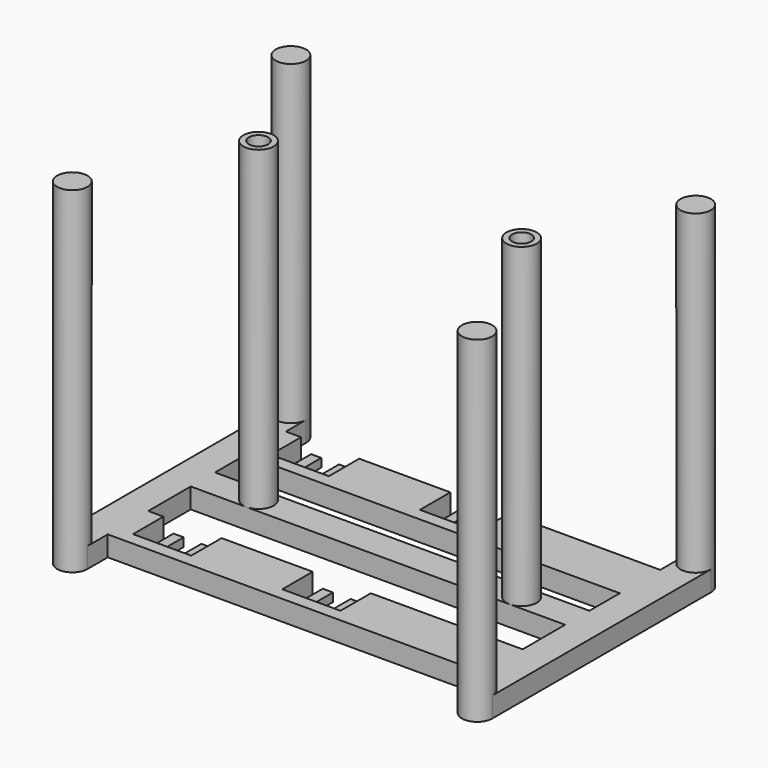
from build123d import *

# Parameters (mm, degrees)
F1_DEPTH  = 4
F2_W      = 2
F2_H      = 7.5
F3_DEPTH  = 1.7
F5_DEPTH  = 62.5
F4_R      = 3
F7_W      = 74
F7_H      = 6
F8_DEPTH  = 4
F9_R      = 1.9
F10_R     = 1.9
F11_DEPTH = 25


with BuildPart() as f1:
    # F0 (on Top) → F1 (new body)
    with BuildSketch(Plane.XY):
        with BuildLine():
            Line((6, 0), (80, 0))
            Line((80, 0), (80, -24))
            Line((80, -24), (80, -34))
            Line((80, -34), (80, -39))
            ThreePointArc((80, -39), (83, -42), (86, -39))
            Line((86, -39), (86, 15))
            ThreePointArc((86, 15), (83, 18), (80, 15))
            Line((80, 15), (80, 10))
            Line((80, 10), (50, 10))
            Line((50, 10), (50, 2.5))
            Line((50, 2.5), (38.5, 2.5))
            Line((38.5, 2.5), (38.5, 10))
            Line((38.5, 10), (20.5, 10))
            Line((20.5, 10), (20.5, 2.5))
            Line((20.5, 2.5), (9, 2.5))
            Line((9, 2.5), (9, 10))
            Line((9, 10), (6, 10))
            Line((6, 10), (6, 15))
            ThreePointArc((6, 15), (3, 18), (0, 15))
            Line((0, 15), (0, -39))
            ThreePointArc((0, -39), (3, -42), (6, -39))
            Line((6, -39), (6, -34))
            Line((6, -34), (6, -24))
            Line((6, -24), (6, 0))
        make_face()
        Polygon((80, -34), (80, -24), (50, -24), (50, -31.5), (38.5, -31.5), (38.5, -24), (20.5, -24), (20.5, -31.5), (9, -31.5), (9, -24), (6, -24), (6, -34), align=None)
    extrude(amount=F1_DEPTH)

    # F2 (on Top) → F3 (join)
    with BuildSketch(Plane.XY):
        with Locations((12, 6.25)):
            Rectangle(F2_W, F2_H)
        with Locations((17.5, 6.25)):
            Rectangle(F2_W, F2_H)
        with Locations((41.5, 6.25)):
            Rectangle(F2_W, F2_H)
        with Locations((47, 6.25)):
            Rectangle(F2_W, F2_H)
        with Locations((12, -27.75)):
            Rectangle(F2_W, F2_H)
        with Locations((17.5, -27.75)):
            Rectangle(F2_W, F2_H)
        with Locations((41.5, -27.75)):
            Rectangle(F2_W, F2_H)
        with Locations((47, -27.75)):
            Rectangle(F2_W, F2_H)
    extrude(amount=F3_DEPTH)

    # F4 (on face) → F5 (join)
    with BuildSketch(Plane.XY.offset(4)):
        with BuildLine():
            ThreePointArc((0, 15), (3, 12), (6, 15))
            ThreePointArc((6, 15), (3, 18), (0, 15))
        make_face()
        with BuildLine():
            ThreePointArc((6, -39), (3, -36), (0, -39))
            ThreePointArc((0, -39), (3, -42), (6, -39))
        make_face()
        with BuildLine():
            ThreePointArc((86, -39), (83, -36), (80, -39))
            ThreePointArc((80, -39), (83, -42), (86, -39))
        make_face()
        with BuildLine():
            ThreePointArc((80, 15), (83, 12), (86, 15))
            ThreePointArc((86, 15), (83, 18), (80, 15))
        make_face()
    extrude(amount=F5_DEPTH)



with BuildPart() as f5:
    # F4 (on face) → F5, piece 2 (new body)
    with BuildSketch(Plane.XY.offset(4)):
        with Locations((17, -10.5)):
            Circle(F4_R)
    extrude(amount=F5_DEPTH)


with BuildPart() as f5b:
    # F4 (on face) → F5, piece 3 (new body)
    with BuildSketch(Plane.XY.offset(4)):
        with Locations((69, -10.5)):
            Circle(F4_R)
    extrude(amount=F5_DEPTH)


with BuildPart() as f1_1:
    add(f1.part)

    add(f5.part)  # F8 merges F5

    add(f5b.part)  # F8 merges F5b
    # F7 (on face) → F8 (join)
    with BuildSketch(Plane(origin=(0, 0, 0), x_dir=(1, 0, 0), z_dir=(0, 0, -1))):
        with Locations((43, 10.5)):
            Rectangle(F7_W, F7_H)
    extrude(amount=-F8_DEPTH)

    # F9 (on face) + F10 (on face) → F11 (cut)
    with BuildSketch(Plane.XY.offset(66.5)):
        with Locations((17, -10.5)):
            Circle(F9_R)
    with BuildSketch(Plane.XY.offset(66.5)):
        with Locations((69, -10.5)):
            Circle(F10_R)
    extrude(amount=-F11_DEPTH, mode=Mode.SUBTRACT)


solid = f1_1.part
